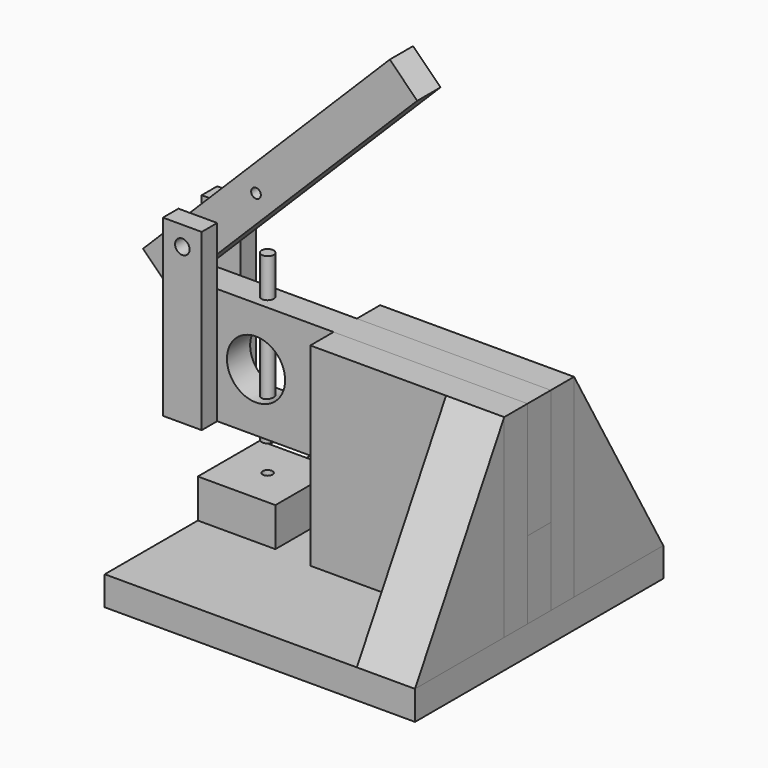
from build123d import *

# Parameters (mm, degrees)
F0_W           = 203.2
F0_H           = 19.05
F1_DEPTH       = 101.6
F2_W           = 127
F2_H           = 50.8
F3_DEPTH       = 9.525
F4_W           = 228.6
F4_H           = 76.2
F5_DEPTH       = 9.525
F6_W           = 127
F6_H           = 127
F7_DEPTH       = 19.05
F10_DEPTH      = 38.1
F12_W          = 50.8
F12_H          = 50.8
F13_DEPTH      = 25.4
F14_R          = 3.175
F15_DEPTH      = 12.7
F16_R          = 4
F17_DEPTH      = 76.2
F18_R          = 19.05
F19_DEPTH      = 111.126
F20_W          = 25.4
F20_H          = 38.1
F20_H_2        = 76.2
F21_DEPTH      = 12.7
F23_R          = 4.7625
F24_DEPTH      = 123.826
F25_R          = 3.175
F26_DEPTH      = 9.525
F27_R          = 4
F28_DEPTH      = 25.4
F28_DEPTH_BACK = 82.55


# Not quite as in the source:
# - a feature names something its author has since deleted; it is built from what else it names


with BuildPart() as f1:
    # F0 (on Front) → F1 (new body, symmetric)
    with BuildSketch(Plane.XZ):
        with Locations((0, 9.525)):
            Rectangle(F0_W, F0_H)
    extrude(amount=F1_DEPTH, both=True)


with BuildPart() as f3:
    # F2 (on Front) → F3 (new body, symmetric)
    with BuildSketch(Plane.XZ):
        with Locations((38.1, 44.45)):
            Rectangle(F2_W, F2_H)
    extrude(amount=F3_DEPTH, both=True)


with BuildPart() as f5:
    # F4 (on Front) → F5 (new body, symmetric)
    with BuildSketch(Plane.XZ):
        with Locations((-12.7, 107.95)):
            Rectangle(F4_W, F4_H)
    extrude(amount=F5_DEPTH, both=True)

    # F16 (on face) → F17 (cut, through all)
    with BuildSketch(Plane.XY.offset(146.05)):
        with Locations((-76.2, 0)):
            Circle(F16_R)
    extrude(amount=-F17_DEPTH, mode=Mode.SUBTRACT)

    # F18 (on face) → F19 (cut, through all)
    with BuildSketch(Plane.XZ.offset(9.525)):
        with Locations((-76.2, 107.95)):
            Circle(F18_R)
    extrude(amount=-F19_DEPTH, mode=Mode.SUBTRACT)


with BuildPart() as f7:
    # F6 (on face) → F7 (new body)
    with BuildSketch(Plane.XZ.offset(9.525)):
        with Locations((38.1, 82.55)):
            Rectangle(F6_W, F6_H)
    extrude(amount=F7_DEPTH)


with BuildPart() as f8_1:
    # F8: instance of F7
    add(f7.part.mirror(Plane.XZ))


with BuildPart() as f10:
    # F9 (on face) → F10 (new body)
    with BuildSketch(Plane.YZ.offset(101.6)):
        Polygon((-28.575, 19.05), (-28.575, 146.05), (-101.6, 19.05), align=None)
    extrude(amount=-F10_DEPTH)


with BuildPart() as f11_1:
    # F11: instance of F10
    add(f10.part.mirror(Plane.XZ))


with BuildPart() as f13:
    # F12 (on face) → F13 (new body)
    with BuildSketch(Plane.XY.offset(19.05)):
        with Locations((-76.2, 0)):
            Rectangle(F12_W, F12_H)
    extrude(amount=F13_DEPTH)

    # F14 (on face) → F15 (cut)
    with BuildSketch(Plane.XY.offset(44.45)):
        with Locations((-76.2, 0)):
            Circle(F14_R)
    extrude(amount=-F15_DEPTH, mode=Mode.SUBTRACT)


with BuildPart() as f21:
    # F20 (on face) → F21 (new body)
    with BuildSketch(Plane.XZ.offset(9.525)):
        with Locations((-114.3, 165.1)):
            Rectangle(F20_W, F20_H)
        with Locations((-114.3, 107.95)):
            Rectangle(F20_W, F20_H_2)
    extrude(amount=F21_DEPTH)


with BuildPart() as f22_1:
    # F22: instance of F21
    add(f21.part.mirror(Plane.XZ))


with BuildPart() as f24_tool:
    # F23 (on face) → F24 (new body, through all)
    with BuildSketch(Plane.XZ.offset(22.225)):
        with Locations((-114.3, 171.45)):
            Circle(F23_R)
    extrude(amount=-F24_DEPTH)


with BuildPart() as f21_1:
    add(f21.part)

    # F24: cut by f24_tool
    add(f24_tool.part, mode=Mode.SUBTRACT)


with BuildPart() as f22_1_1:
    add(f22_1.part)

    # F24: cut by f24_tool
    add(f24_tool.part, mode=Mode.SUBTRACT)


with BuildPart() as f26:
    # F25 (on Front) → F26 (new body, symmetric)
    with BuildSketch(Plane.XZ):
        Polygon((-150.2210244843, 153.4894877579), (-132.2605122421, 135.5289755157), (29.3840979371, 297.173585695), (11.423585695, 315.1340979371), align=None)
        with BuildLine():
            ThreePointArc((-117.6675960454, 174.8175960454), (-110.9324039546, 174.8175960454), (-110.9324039546, 168.0824039546))
            Line((-110.9324039546, 168.0824039546), (-124.4027881362, 154.612019773))
            ThreePointArc((-124.4027881362, 154.612019773), (-131.137980227, 154.612019773), (-131.137980227, 161.3472118638))
            Line((-131.137980227, 161.3472118638), (-117.6675960454, 174.8175960454))
        make_face(mode=Mode.SUBTRACT)
        with Locations((-76.2, 209.55)):
            Circle(F25_R, mode=Mode.SUBTRACT)
    extrude(amount=F26_DEPTH, both=True)


with BuildPart() as f28:
    # F27 (on face) → F28 (new body, two sides)
    with BuildSketch(Plane.XY.offset(146.05)) as f28_sk:
        with Locations((-76.2, 0)):
            Circle(F27_R)
    extrude(amount=F28_DEPTH)
    extrude(f28_sk.sketch, amount=-F28_DEPTH_BACK)


solid = Compound([f1.part, f3.part, f5.part, f7.part, f8_1.part, f10.part, f11_1.part, f13.part, f21_1.part, f22_1_1.part, f26.part, f28.part])
